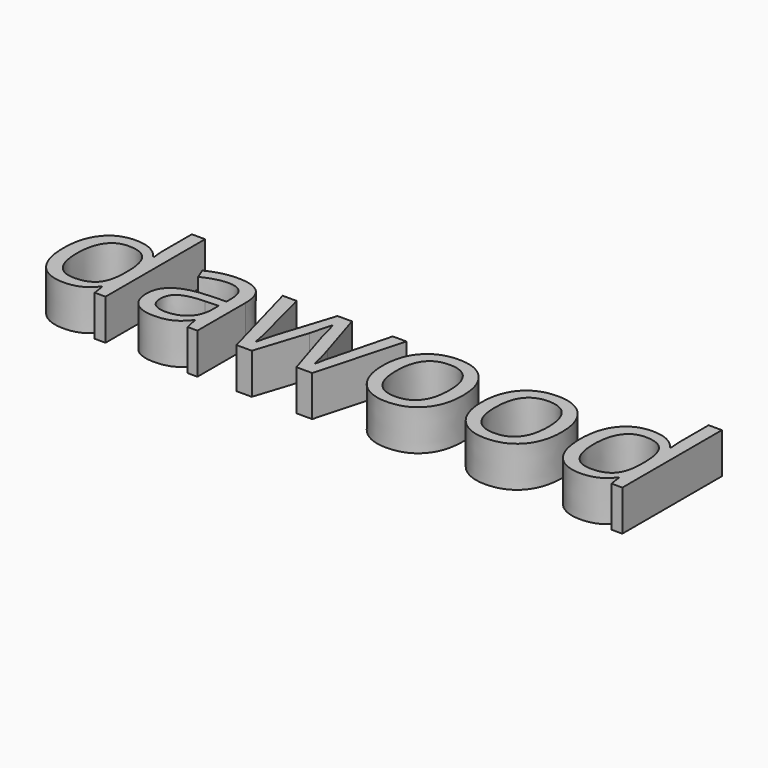
from build123d import *

# Parameters (mm, degrees)
F0_TEXT_SIZE = 20.1690176408
F1_DEPTH     = 5


# Not quite as in the source:
# - Text() gives the source's letters only with a copy of the font that has no kerning and outlines rounded to 1/6400 em; it was checked with that copy


with BuildPart() as f1:
    # F0 (on Top) → F1 (new body)
    with BuildSketch(Plane.XY):
        with Locations((0, 0)):
            Text('dawood', F0_TEXT_SIZE, font='Open Sans', text_align=(TextAlign.LEFT, TextAlign.BOTTOM))
    extrude(amount=F1_DEPTH)


solid = f1.part
